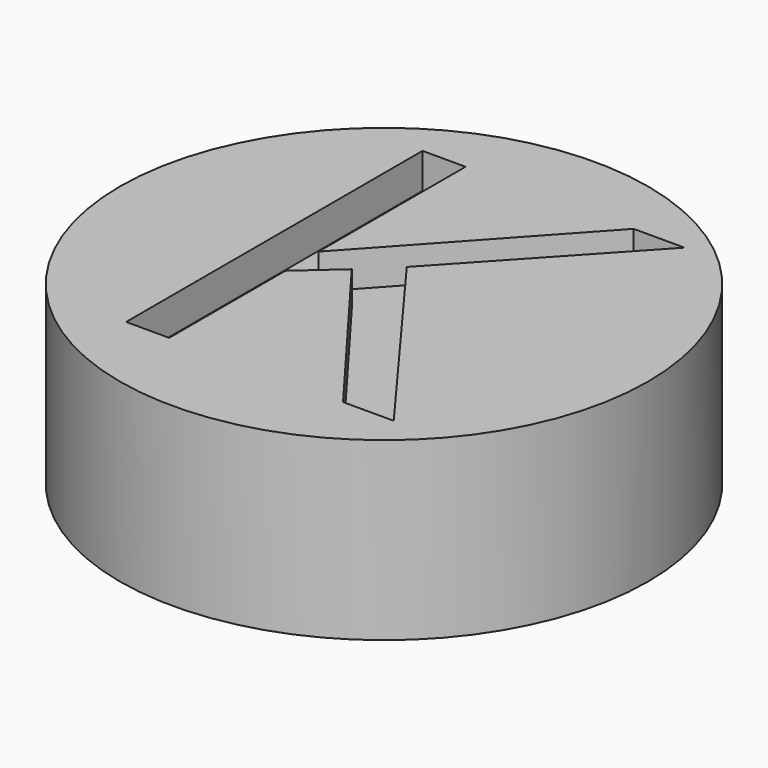
from build123d import *

# Parameters (mm, degrees)
F0_R         = 19.05
F1_DEPTH     = 12.7
F3_START     = 10.16
F2_TEXT_SIZE = 37.4303476859
F3_DEPTH     = 2.54


# Not quite as in the source:
# - Text() gives the source's letters only with a copy of the font that has no kerning and outlines rounded to 1/6400 em; it was checked with that copy


with BuildPart() as f1:
    # F0 (on Top) → F1 (new body)
    with BuildSketch(Plane.XY):
        Circle(F0_R)
    extrude(amount=F1_DEPTH)

    # F2 (on Top) → F3 (cut)
    with BuildSketch(Plane.XY.offset(F3_START)):
        with Locations((-12.1238188387, -12.6869230024)):
            Text('K', F2_TEXT_SIZE, font='Open Sans', text_align=(TextAlign.LEFT, TextAlign.BOTTOM))
    extrude(amount=F3_DEPTH, mode=Mode.SUBTRACT)


solid = f1.part
